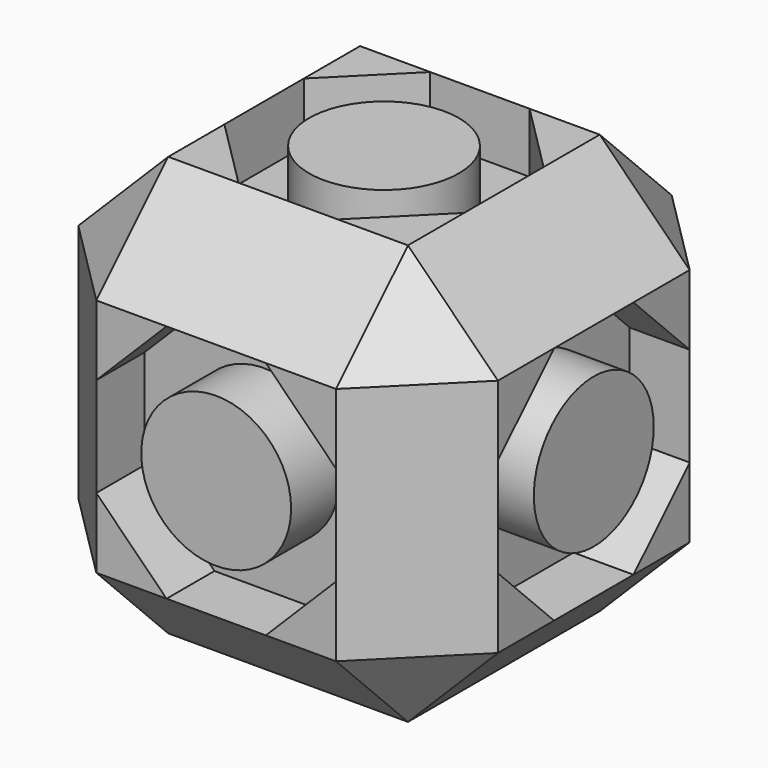
from build123d import *

# Parameters (mm, degrees)
F0_W      = 14
F0_H      = 14
F1_DEPTH  = 7
F2_R      = 2.5
F4_DEPTH  = 2
F5_SIZE   = 2.99999
F6_R      = 2.5
F11_DEPTH = 2
F7_R      = 2.5
F12_DEPTH = 2
F8_R      = 2.5
F13_DEPTH = 2
F9_R      = 2.5
F14_DEPTH = 2
F10_R     = 2.5
F15_DEPTH = 2


# Not quite as in the source:
# - a fillet or chamfer is up to 0.001 mm smaller than in the source, because OpenCascade refuses the exact size


with BuildPart() as f1:
    # F0 (on Top) → F1 (new body, symmetric)
    with BuildSketch(Plane.XY):
        Rectangle(F0_W, F0_H)
    extrude(amount=F1_DEPTH, both=True)

    # F2 (on face) → F4 (cut)
    with BuildSketch(Plane.YZ.offset(7)):
        Polygon((-4, 1.6568542495), (-4, -1.6568542495), (-1.6568542495, -4), (1.6568542495, -4), (4, -1.6568542495), (4, 1.6568542495), (1.6568542495, 4), (-1.6568542495, 4), align=None)
        Circle(F2_R, mode=Mode.SUBTRACT)
    extrude(amount=-F4_DEPTH, mode=Mode.SUBTRACT)

    # F5 (size 3 in the source; OpenCascade refuses exactly that, so slightly less here)
    f5_edges = [f1.edges().sort_by_distance(p)[0] for p in [
        (7, 7, 0),
        (0, 7, -7),
        (-7, 7, 0),
        (0, 7, 7),
        (0, -7, 7),
        (7, 0, 7),
        (-7, 0, 7),
        (0, -7, -7),
        (7, -7, 0),
        (-7, -7, 0),
        (7, 0, -7),
        (-7, 0, -7),
    ]]
    chamfer(f5_edges, length=F5_SIZE)

    # F6 (on face) → F11 (cut)
    with BuildSketch(Plane(origin=(0, 7, 0), x_dir=(-1, 0, 0), z_dir=(0, 1, 0))):
        Polygon((-4, 1.6568542495), (-4, -1.6568542495), (-1.6568542495, -4), (1.6568542495, -4), (4, -1.6568542495), (4, 1.6568542495), (1.6568542495, 4), (-1.6568542495, 4), align=None)
        Circle(F6_R, mode=Mode.SUBTRACT)
    extrude(amount=-F11_DEPTH, mode=Mode.SUBTRACT)

    # F7 (on face) → F12 (cut)
    with BuildSketch(Plane.XY.offset(7)):
        Polygon((-4, 1.6568542495), (-4, -1.6568542495), (-1.6568542495, -4), (1.6568542495, -4), (4, -1.6568542495), (4, 1.6568542495), (1.6568542495, 4), (-1.6568542495, 4), align=None)
        Circle(F7_R, mode=Mode.SUBTRACT)
    extrude(amount=-F12_DEPTH, mode=Mode.SUBTRACT)

    # F8 (on face) → F13 (cut)
    with BuildSketch(Plane(origin=(-7, 0, 0), x_dir=(0, -1, 0), z_dir=(-1, 0, 0))):
        Polygon((-4, 1.6568542495), (-4, -1.6568542495), (-1.6568542495, -4), (1.6568542495, -4), (4, -1.6568542495), (4, 1.6568542495), (1.6568542495, 4), (-1.6568542495, 4), align=None)
        Circle(F8_R, mode=Mode.SUBTRACT)
    extrude(amount=-F13_DEPTH, mode=Mode.SUBTRACT)

    # F9 (on face) → F14 (cut)
    with BuildSketch(Plane.XZ.offset(7)):
        Polygon((-4, 1.6568542495), (-4, -1.6568542495), (-1.6568542495, -4), (1.6568542495, -4), (4, -1.6568542495), (4, 1.6568542495), (1.6568542495, 4), (-1.6568542495, 4), align=None)
        Circle(F9_R, mode=Mode.SUBTRACT)
    extrude(amount=-F14_DEPTH, mode=Mode.SUBTRACT)

    # F10 (on face) → F15 (cut)
    with BuildSketch(Plane(origin=(0, 0, -7), x_dir=(1, 0, 0), z_dir=(0, 0, -1))):
        Polygon((-4, 1.6568542495), (-4, -1.6568542495), (-1.6568542495, -4), (1.6568542495, -4), (4, -1.6568542495), (4, 1.6568542495), (1.6568542495, 4), (-1.6568542495, 4), align=None)
        Circle(F10_R, mode=Mode.SUBTRACT)
    extrude(amount=-F15_DEPTH, mode=Mode.SUBTRACT)


solid = f1.part
